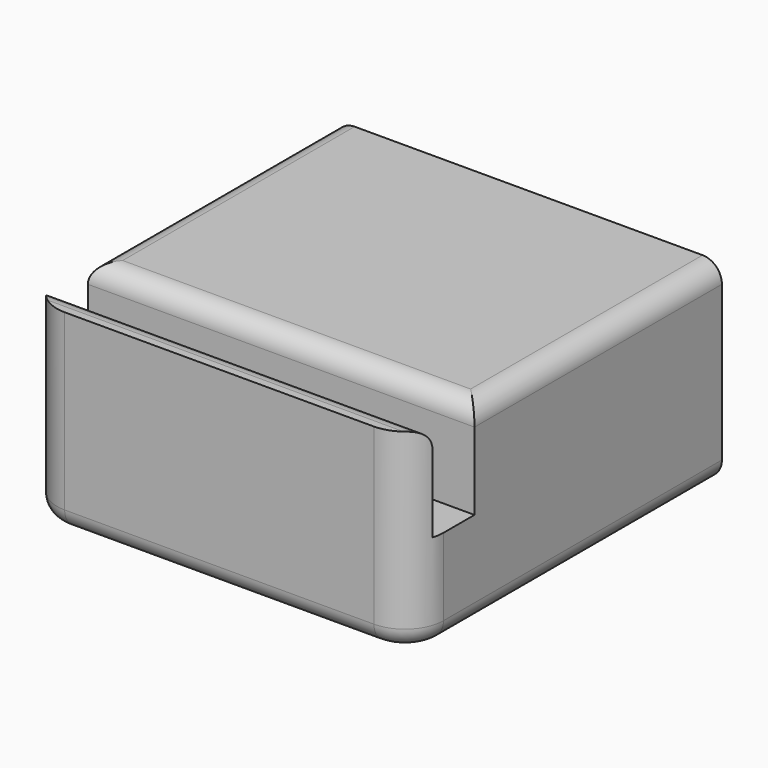
from build123d import *

# Parameters (mm, degrees)
F1_DEPTH    = 10
F2_W        = 4.5836600475
F2_H        = 4
F3_DEPTH    = 25
F4_W        = 2.6
F4_H        = 5
F5_DEPTH    = 25
F6_R        = 3
F7_R        = 3
F8_R        = 1
F9_T1_DEPTH = 15
F9_T4_ANGLE = 90
F9_T6_ANGLE = 90


# Not quite as in the source:
# - a fillet or chamfer that OpenCascade refuses, or shapes differently, is made with other operations: its cross-section is extruded or revolved along the edge and cut away or added


with BuildPart() as f1:
    # F0 (on Top) → F1 (new body)
    with BuildSketch(Plane.XY):
        Polygon((4.5, 4), (0, 4), (-4.5, 4), (-4.5, 1), (-3, 1), (-3, 0), (-4.5, 0), (-10, 0), (-10, -20), (0, -20), (10, -20), (10, 0), (4.5, 0), (3, 0), (3, 1), (4.5, 1), align=None)
    extrude(amount=F1_DEPTH)

    # F2 (on face) → F3 (cut)
    with BuildSketch(Plane(origin=(-10, 0, 0), x_dir=(0, -1, 0), z_dir=(-1, 0, 0))):
        with Locations((-2.2918300238, 8)):
            Rectangle(F2_W, F2_H)
    extrude(amount=-F3_DEPTH, mode=Mode.SUBTRACT)

    # F4 (on face) → F5 (cut)
    with BuildSketch(Plane.YZ.offset(10)):
        with Locations((-17.3, 7.5)):
            Rectangle(F4_W, F4_H)
    extrude(amount=-F5_DEPTH, mode=Mode.SUBTRACT)

    # F6
    f6_edges = [f1.edges().sort_by_distance(p)[0] for p in [
        (3, 0.5, 0),
        (-3, 0.5, 6),
    ]]
    fillet(f6_edges, radius=F6_R)

    # F7
    f7_edges = [f1.edges().sort_by_distance(p)[0] for p in [
        (4.5, 2.5, 0),
        (-4.5, 2.5, 6),
    ]]
    fillet(f7_edges, radius=F7_R)

    # F8
    f8_edges = [f1.edges().sort_by_distance(p)[0] for p in [
        (-10, -8, 10),
        (10, -8, 10),
        (-10, -10, 0),
        (0, -20, 0),
        (10, -10, 0),
        (0, -18.6, 10),
        (0, -16, 10),
    ]]
    fillet(f8_edges, radius=F8_R)

    # F9: fillet of radius 2 on 2 edges, made by hand

    # F9_s2 → F9_t1 (cut)
    with BuildSketch(Plane.XY):
        with BuildLine():
            ThreePointArc((10, -18), (9.4142135624, -19.4142135624), (8, -20))
            Line((8, -20), (10, -20))
            Line((10, -20), (10, -18))
        make_face()
        with BuildLine():
            ThreePointArc((-10, -18), (-9.4142135624, -19.4142135624), (-8, -20))
            Line((-8, -20), (-10, -20))
            Line((-10, -20), (-10, -18))
        make_face()
    extrude(amount=F9_T1_DEPTH, mode=Mode.SUBTRACT)

    # F9_s3 → F9_t4 (revolve, cut)
    with BuildSketch(Plane.YZ.offset(-8)):
        with BuildLine():
            ThreePointArc((-19, 0), (-19.7071067812, 0.2928932188), (-20, 1))
            Line((-20, 1), (-20, 0))
            Line((-20, 0), (-19, 0))
        make_face()
    revolve(axis=Axis((-8, -18, 0), (0, 0, -1)), revolution_arc=F9_T4_ANGLE, mode=Mode.SUBTRACT)

    # F9_s5 → F9_t6 (revolve, cut)
    with BuildSketch(Plane.XZ.offset(18)):
        with BuildLine():
            ThreePointArc((9, 0), (9.7071067812, 0.2928932188), (10, 1))
            Line((10, 1), (10, 0))
            Line((10, 0), (9, 0))
        make_face()
    revolve(axis=Axis((8, -18, 0), (0, 0, -1)), revolution_arc=F9_T6_ANGLE, mode=Mode.SUBTRACT)


solid = f1.part
